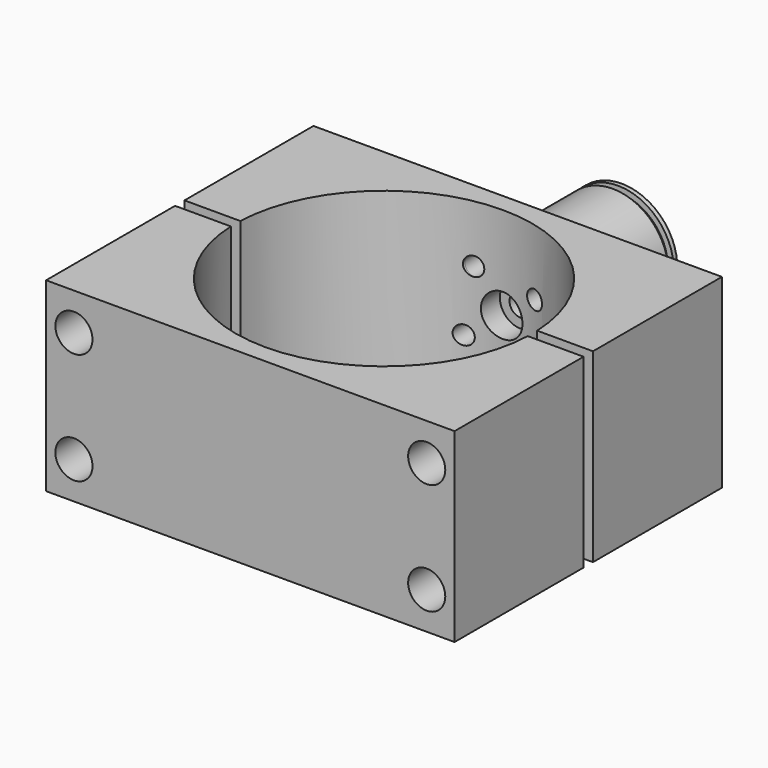
from build123d import *

# Parameters (mm, degrees)
F0_R           = 14.99619
F0_R_2         = 6.36016
F1_DEPTH       = 35
F2_W           = 110
F2_H           = 50
F3_DEPTH       = 90
F4_R           = 5
F5_DEPTH       = 70
F7_DEPTH       = 50.001
F8_R           = 14.99619
F8_R_2         = 13.4493
F9_DEPTH       = 3
F10_R          = 14.99619
F10_R_2        = 13.4493
F11_DEPTH      = 1.22174
F12_R          = 16.99619
F12_R_2        = 14.99619
F13_DEPTH      = 4
F14_R          = 7.8345578302
F15_DEPTH      = 6
F16_R          = 3
F17_DEPTH      = 25
F19_R          = 5.6
F20_DEPTH      = 6.5
F19_R_2        = 2.5
F21_DEPTH      = 15
F21_DEPTH_BACK = 25


# Not quite as in the source:
# - a feature names something its author has since deleted; it is built from what else it names


with BuildPart() as f1:
    # F0 (on Front) → F1 (new body)
    with BuildSketch(Plane.XZ):
        Circle(F0_R)
        Circle(F0_R_2, mode=Mode.SUBTRACT)
    extrude(amount=F1_DEPTH)

    # F2 (on face) → F3 (join)
    with BuildSketch(Plane.XZ.offset(35)):
        Rectangle(F2_W, F2_H)
    extrude(amount=F3_DEPTH)

    # F4 (on face) → F5 (cut)
    with BuildSketch(Plane.XZ.offset(125)):
        with Locations((-47.5, 15)):
            Circle(F4_R)
        with Locations((-47.5, -15)):
            Circle(F4_R)
        with Locations((47.5, 15)):
            Circle(F4_R)
        with Locations((47.5, -15)):
            Circle(F4_R)
    extrude(amount=-F5_DEPTH, mode=Mode.SUBTRACT)

    # F6 (on face) → F7 (cut, through all)
    with BuildSketch(Plane.XY.offset(25)):
        with BuildLine():
            Line((-58.9964538813, -81.5874989), (-39.9684856761, -81.5874989))
            ThreePointArc((-39.9684856761, -81.5874989), (0, -120), (39.9684856761, -81.5874989))
            Line((39.9684856761, -81.5874989), (59.7361437976, -81.5874989))
            Line((59.7361437976, -81.5874989), (59.7361437976, -78.4124989))
            Line((59.7361437976, -78.4124989), (39.9684855887, -78.4124989))
            ThreePointArc((39.9684855887, -78.4124989), (0, -40), (-39.9684855887, -78.4124989))
            Line((-39.9684855887, -78.4124989), (-58.9964538813, -78.4124989))
            Line((-58.9964538813, -78.4124989), (-58.9964538813, -81.5874989))
        make_face()
    extrude(amount=-F7_DEPTH, mode=Mode.SUBTRACT)

    # F8 (on face) → F9 (cut)
    with BuildSketch(Plane(origin=(0, 0, 0), x_dir=(-1, 0, 0), z_dir=(0, 1, 0))):
        Circle(F8_R)
        Circle(F8_R_2, mode=Mode.SUBTRACT)
    extrude(amount=-F9_DEPTH, mode=Mode.SUBTRACT)

    # F10 (on face) → F11 (join)
    with BuildSketch(Plane(origin=(0, 0, 0), x_dir=(-1, 0, 0), z_dir=(0, 1, 0))):
        Circle(F10_R)
        Circle(F10_R_2, mode=Mode.SUBTRACT)
    extrude(amount=-F11_DEPTH)

    # F12 (on face) → F13 (join)
    with BuildSketch(Plane(origin=(0, -35, 0), x_dir=(-1, 0, 0), z_dir=(0, 1, 0))):
        Circle(F12_R)
        Circle(F12_R_2, mode=Mode.SUBTRACT)
    extrude(amount=F13_DEPTH)

    # F14 (on face) → F15 (join)
    with BuildSketch(Plane(origin=(0, -35, 0), x_dir=(-1, 0, 0), z_dir=(0, 1, 0))):
        Circle(F14_R)
    extrude(amount=F15_DEPTH)

    # F16 (on face) → F17 (cut)
    with BuildSketch(Plane(origin=(0, -29, 0), x_dir=(-1, 0, 0), z_dir=(0, 1, 0))):
        Circle(F16_R)
    extrude(amount=-F17_DEPTH, mode=Mode.SUBTRACT)

    # F19 (on offset) → F20 (cut)
    with BuildSketch(Plane.XZ.offset(40.5)):
        Circle(F19_R)
    extrude(amount=-F20_DEPTH, mode=Mode.SUBTRACT)

    # F19 (on offset) → F21 (cut, two sides)
    with BuildSketch(Plane.XZ.offset(40.5)) as f21_sk:
        with Locations((7.2691551531, -9.5426725713)):
            Circle(F19_R_2)
        with Locations((9.5429855552, 7.2691128213)):
            Circle(F19_R_2)
        with Locations((-7.2687998374, 9.5429432235)):
            Circle(F19_R_2)
        with Locations((-9.5426302396, -7.2688421692)):
            Circle(F19_R_2)
    extrude(amount=-F21_DEPTH, mode=Mode.SUBTRACT)
    extrude(f21_sk.sketch, amount=F21_DEPTH_BACK, mode=Mode.SUBTRACT)


solid = f1.part
